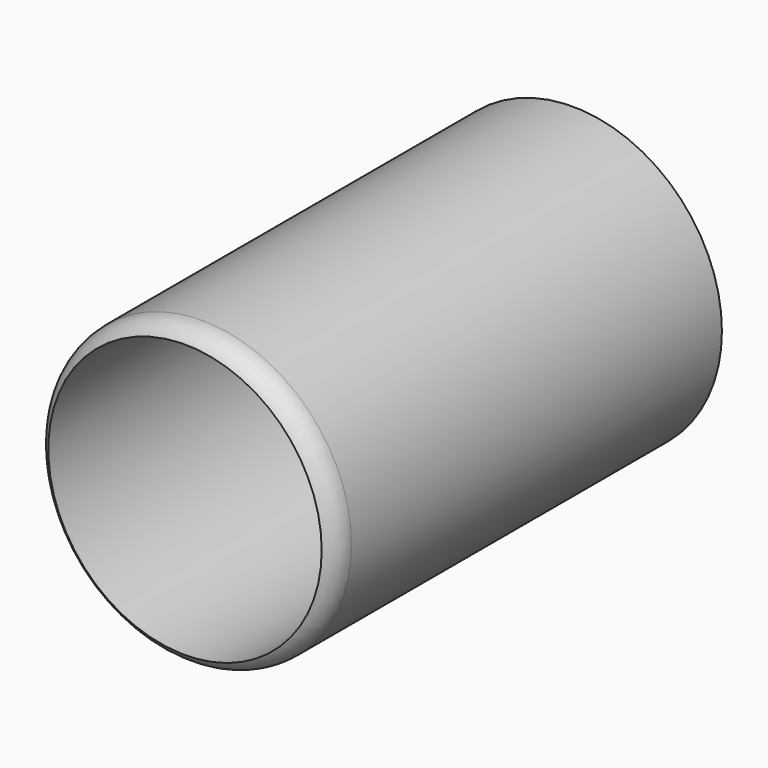
from build123d import *

# Parameters (mm, degrees)
F0_R     = 34.925
F1_DEPTH = 9.525
F0_R_2   = 38.1
F2_DEPTH = 123.825


# Not quite as in the source:
# - a fillet or chamfer that OpenCascade refuses, or shapes differently, is made with other operations: its cross-section is extruded or revolved along the edge and cut away or added


with BuildPart() as f1:
    # F0 (on Front) → F1 (new body)
    with BuildSketch(Plane.XZ):
        Circle(F0_R)
    extrude(amount=F1_DEPTH)

    # F0 (on Front) → F2 (join)
    with BuildSketch(Plane.XZ):
        Circle(F0_R_2)
        Circle(F0_R, mode=Mode.SUBTRACT)
    extrude(amount=F2_DEPTH)

    # F3: fillet of radius 6.35 on 1 edges, made by hand

    # F3_s1 → F3_t2 (revolve, cut)
    with BuildSketch(Plane.XY):
        with BuildLine():
            ThreePointArc((38.1, -118.325738686), (37.249261314, -121.500738686), (34.925, -123.825))
            Line((34.925, -123.825), (38.1, -123.825))
            Line((38.1, -123.825), (38.1, -118.325738686))
        make_face()
    revolve(axis=Axis((0, -123.825, 0), (0, -1, 0)), mode=Mode.SUBTRACT)


solid = f1.part
